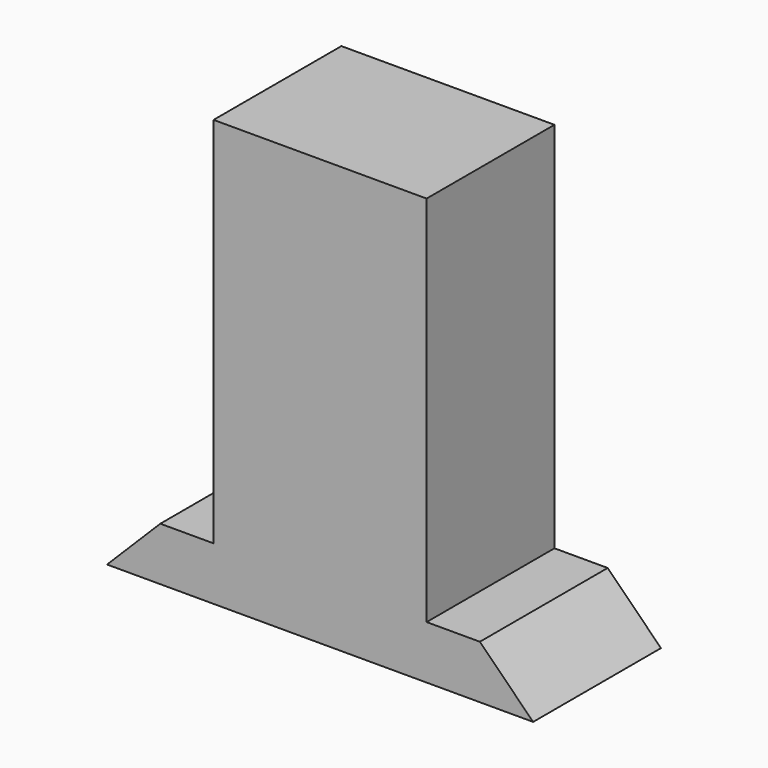
from build123d import *

# Parameters (mm, degrees)
F0_W      = 80
F0_H      = 30
F1_DEPTH  = 10
F2_SIZE   = 9.99999
F4_DEPTH  = 40
F4_FACE_W = 40
F4_FACE_H = 30
F5_DEPTH  = 40


# Not quite as in the source:
# - a fillet or chamfer is up to 0.001 mm smaller than in the source, because OpenCascade refuses the exact size


with BuildPart() as f1:
    # F0 (on Top) → F1 (new body)
    with BuildSketch(Plane.XY):
        Rectangle(F0_W, F0_H)
    extrude(amount=F1_DEPTH)

    # F2 (size 10 in the source; OpenCascade refuses exactly that, so slightly less here)
    f2_edges = [f1.edges().sort_by_distance(p)[0] for p in [
        (40, 0, 10),
        (-40, 0, 10),
    ]]
    chamfer(f2_edges, length=F2_SIZE)

    # F3 (on Top) → F4 (join)
    with BuildSketch(Plane.XY):
        Polygon((20, -15), (20, 15), (16.5369563365, -15), align=None)
        Polygon((16.5369563365, -15), (20, 15), (-16.5369563365, 15), (-20, -15), align=None)
        Polygon((-20, -15), (-16.5369563365, 15), (-20, 15), align=None)
    extrude(amount=F4_DEPTH)

    # F3 (on Top) + F4_face (on face) → F5 (join)
    with BuildSketch(Plane.XY):
        Polygon((20, -15), (20, 15), (16.5369563365, -15), align=None)
        Polygon((16.5369563365, -15), (20, 15), (-16.5369563365, 15), (-20, -15), align=None)
        Polygon((-20, -15), (-16.5369563365, 15), (-20, 15), align=None)
    with BuildSketch(Plane.XY.offset(40)):
        Rectangle(F4_FACE_W, F4_FACE_H)
    extrude(amount=F5_DEPTH)


solid = f1.part
